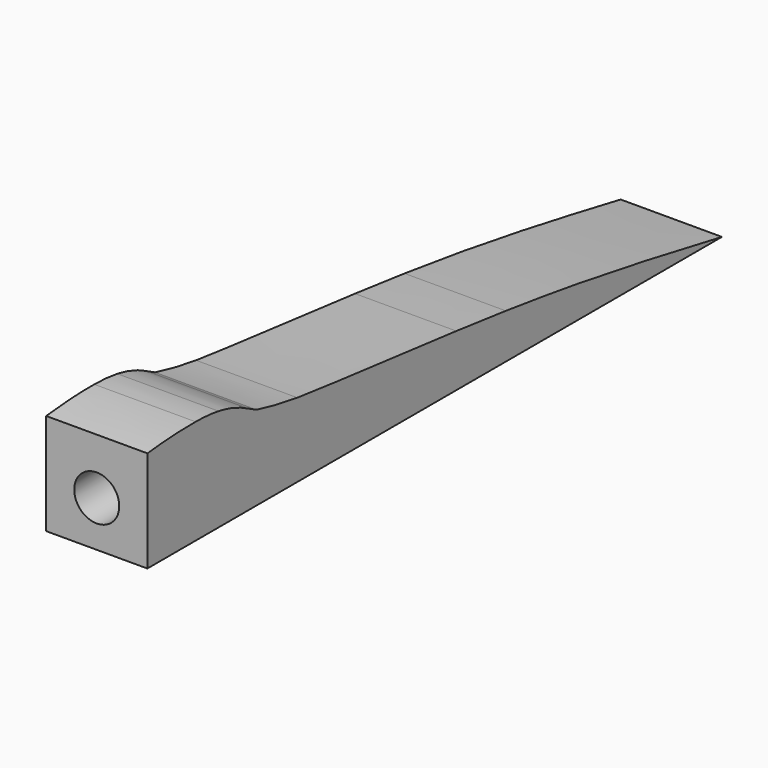
from build123d import *

# Parameters (mm, degrees)
F1_DEPTH = 21.43125
F2_R     = 9.525
F3_DEPTH = 50.8
F8_DEPTH = 56.3


# Not quite as in the source:
# - ends of sketch curves that miss each other by under 0.0002 mm in the source are joined


with BuildPart() as f1:
    # F0 (on Right) → F1 (new body, symmetric)
    with BuildSketch(Plane.YZ):
        Polygon((-152.4, 69.85), (-152.4, 0), (152.4, 0), (152.4, 19.05), align=None)
    extrude(amount=F1_DEPTH, both=True)

    # F2 (on face) → F3 (cut)
    with BuildSketch(Plane.XZ.offset(152.4)):
        with Locations((0, 34.925)):
            Circle(F2_R)
    extrude(amount=-F3_DEPTH, mode=Mode.SUBTRACT)

    # F5 (on face) → F8 (cut)
    with BuildSketch(Plane.YZ.offset(21.43125)):
        with BuildLine():
            add(Edge.make_bspline(
                [(-94.6281477809, 51.2691959739), (-96.0952206694, 52.0179937663), (-97.562293558, 52.7667915588), (-99.0539994454, 53.491879309)],
                knots=[0, 0, 0, 0, 0.1035282224, 0.1035282224, 0.1035282224, 0.1035282224], degree=3))
            add(Edge.make_bspline(
                [(-94.6281477809, 51.2691959739), (-88.9739529123, 49.8775010567), (-83.3197580522, 48.4858061416), (-73.0600804397, 46.9911508307)],
                knots=[0, 0, 0, 0, 0.1804237123, 0.1804237123, 0.1804237123, 0.1804237123], degree=3))
            add(Edge.make_bspline(
                [(11.0397725003, 37.6377859426), (-20.7191231776, 41.240284312), (-53.8117553476, 44.4768553148), (-73.0600804397, 46.9911508307)],
                knots=[0.3821429542, 0.3821429542, 0.3821429542, 0.3821429542, 0.5639196837, 0.5639196837, 0.5639196837, 0.5639196837], degree=3))
            add(Edge.make_bspline(
                [(11.0397725003, 37.6377859426), (19.8326583687, 36.6506728683), (28.6537852654, 35.611343032), (37.2394360057, 34.5120057533)],
                knots=[0.5008053198, 0.5008053198, 0.5008053198, 0.5008053198, 0.5858071806, 0.5858071806, 0.5858071806, 0.5858071806], degree=3))
            add(Edge.make_bspline(
                [(151.5644788742, 15.5920218676), (140.3358248303, 17.736038831), (112.6697575345, 23.0186414795), (69.4706003693, 30.4232191611), (37.2394360057, 34.5120057533)],
                knots=[0, 0, 0, 0, 0.1343010577, 0.3309018237, 0.3309018237, 0.3309018237, 0.3309018237], degree=3))
            Line((151.5644788742, 15.5920218676), (-152.4, 15.5920218676))
            Line((-152.4, 15.5920218676), (-152.4, 0))
            Line((-152.4, 0), (152.4, 0))
            Line((152.4, 0), (152.4, 19.05))
            Line((152.4, 19.05), (-152.4, 69.85))
            Line((-152.4, 69.85), (-152.4, 58.510940522))
            add(Edge.make_bspline(
                [(-152.1597802639, 58.510940522), (-152.2398342689, 58.510940522), (-152.3198882739, 58.510940522), (-152.4, 58.510940522)],
                knots=[0, 0, 0, 0, 0.240162015, 0.240162015, 0.240162015, 0.240162015], degree=3))
            add(Edge.make_bspline(
                [(-126.880271242, 59.893312547), (-131.0252775202, 59.9641176604), (-141.283309107, 59.6280745769), (-148.0759439731, 58.9303957414), (-152.1597802639, 58.510940522)],
                knots=[0.8645812396, 0.8645812396, 0.8645812396, 0.8645812396, 0.9185841637, 1, 1, 1, 1], degree=3))
            add(Edge.make_bspline(
                [(-114.7441045161, 58.9132569857), (-118.4444301689, 59.5720764958), (-122.5362126789, 59.8541063708), (-126.880271242, 59.893312547)],
                knots=[0.431288265, 0.431288265, 0.431288265, 0.431288265, 0.6334912794, 0.6334912794, 0.6334912794, 0.6334912794], degree=3))
            add(Edge.make_bspline(
                [(-99.0539994454, 53.491879309), (-99.5844007901, 53.7839672826), (-103.1690308471, 55.7243154808), (-108.8461739052, 57.9235356565), (-114.7441045161, 58.9132569857)],
                knots=[0.7100922868, 0.7100922868, 0.7100922868, 0.7100922868, 0.7255634136, 0.8104095628, 0.8104095628, 0.8104095628, 0.8104095628], degree=3))
        make_face()
    extrude(amount=-F8_DEPTH, mode=Mode.SUBTRACT)


solid = f1.part
